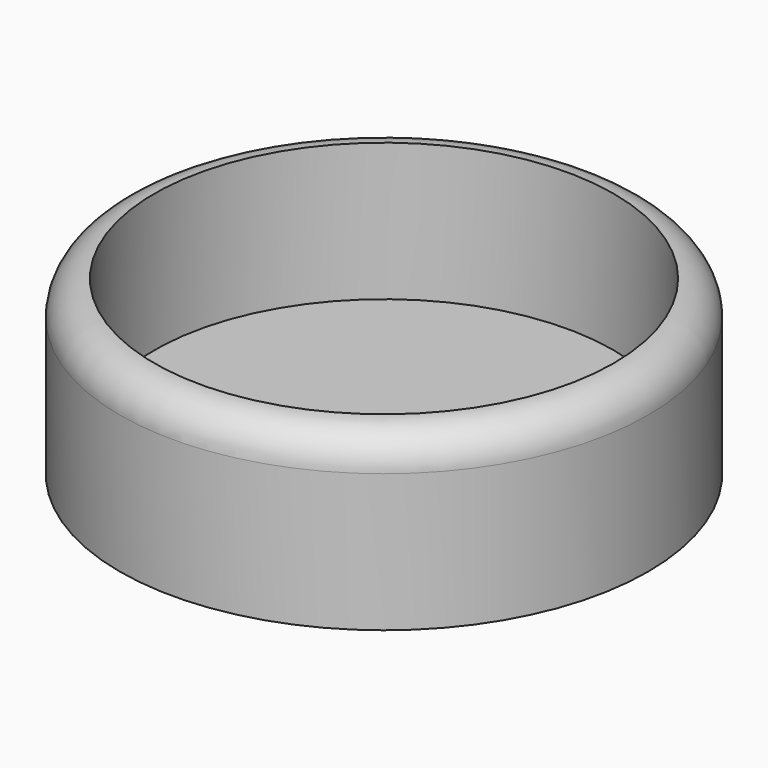
from build123d import *

# Parameters (mm, degrees)
F0_R     = 23
F0_R_2   = 20
F1_DEPTH = 15
F2_R     = 23
F3_DEPTH = 3
F4_R     = 2.99999


# Not quite as in the source:
# - a fillet or chamfer is up to 0.001 mm smaller than in the source, because OpenCascade refuses the exact size


with BuildPart() as f1:
    # F0 (on Top) → F1 (new body)
    with BuildSketch(Plane.XY):
        Circle(F0_R)
        Circle(F0_R_2, mode=Mode.SUBTRACT)
    extrude(amount=F1_DEPTH)

    # F2 (on Top) → F3 (join)
    with BuildSketch(Plane.XY):
        Circle(F2_R)
    extrude(amount=F3_DEPTH)

    # F4 (radius 3 in the source; OpenCascade refuses exactly that, so slightly less here)
    f4_edges = [f1.edges().sort_by_distance(p)[0] for p in [
        (-23, 0, 15),
    ]]
    fillet(f4_edges, radius=F4_R)


solid = f1.part
